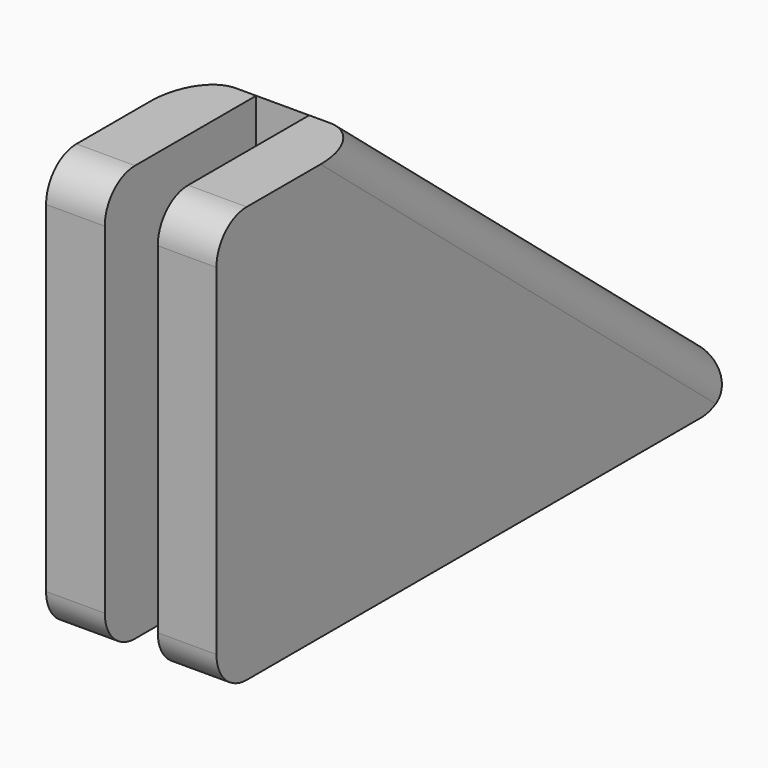
from build123d import *

# Parameters (mm, degrees)
F0_W     = 5
F0_H     = 10
F1_DEPTH = 4.5
F2_W     = 1.4
F2_H     = 5
F3_DEPTH = 25
F4_W     = 1.4
F4_H     = 1
F5_DEPTH = 25
F6_R     = 0.99999
F6_R_2   = 1
F7_R     = 5


# Not quite as in the source:
# - a fillet or chamfer is up to 0.001 mm smaller than in the source, because OpenCascade refuses the exact size


with BuildPart() as f1:
    # F0 (on Right) → F1 (new body)
    with BuildSketch(Plane.YZ):
        with Locations((-2.5, 5)):
            Rectangle(F0_W, F0_H)
        Polygon((0, 10), (0, 0), (12, 0), align=None)
        Polygon((12, 0), (0, 0), (-5, 0), (-5, -1), (12, -1), align=None)
    extrude(amount=F1_DEPTH)

    # F2 (on face) → F3 (cut)
    with BuildSketch(Plane.XY.offset(10)):
        with Locations((2.25, -2.5)):
            Rectangle(F2_W, F2_H)
    extrude(amount=-F3_DEPTH, mode=Mode.SUBTRACT)

    # F4 (on face) → F5 (cut)
    with BuildSketch(Plane(origin=(0, 12, 0), x_dir=(-1, 0, 0), z_dir=(0, 1, 0))):
        with Locations((-2.25, -0.5)):
            Rectangle(F4_W, F4_H)
    extrude(amount=-F5_DEPTH, mode=Mode.SUBTRACT)

    # F6 (call 1 of 8: OpenCascade refuses the feature's edges together) (radius 1 in the source; OpenCascade refuses exactly that, so slightly less here)
    f6_edges = [f1.edges().sort_by_distance(p)[0] for p in [
        (3.725, 12, -1),
    ]]
    fillet(f6_edges, radius=F6_R)

    # F6#2 (call 2 of 8) (radius 1 in the source; OpenCascade refuses exactly that, so slightly less here)
    f6_2_edges = [f1.edges().sort_by_distance(p)[0] for p in [
        (0.775, 12, -1),
    ]]
    fillet(f6_2_edges, radius=F6_R)

    # F6#3 (call 3 of 8)
    f6_3_edges = [f1.edges().sort_by_distance(p)[0] for p in [
        (3.725, -5, -1),
    ]]
    fillet(f6_3_edges, radius=F6_R_2)

    # F6#4 (call 4 of 8)
    f6_4_edges = [f1.edges().sort_by_distance(p)[0] for p in [
        (0.775, -5, -1),
    ]]
    fillet(f6_4_edges, radius=F6_R_2)

    # F6#5 (call 5 of 8)
    f6_5_edges = [f1.edges().sort_by_distance(p)[0] for p in [
        (0.775, -5, 10),
    ]]
    fillet(f6_5_edges, radius=F6_R_2)

    # F6#6 (call 6 of 8)
    f6_6_edges = [f1.edges().sort_by_distance(p)[0] for p in [
        (3.725, -5, 10),
    ]]
    fillet(f6_6_edges, radius=F6_R_2)

    # F6#7 (call 7 of 8)
    f6_7_edges = [f1.edges().sort_by_distance(p)[0] for p in [
        (0, 6, 5),
    ]]
    fillet(f6_7_edges, radius=F6_R_2)

    # F6#8 (call 8 of 8)
    f6_8_edges = [f1.edges().sort_by_distance(p)[0] for p in [
        (4.5, 6, 5),
    ]]
    fillet(f6_8_edges, radius=F6_R_2)

    # F7
    f7_edges = [f1.edges().sort_by_distance(p)[0] for p in [
        (2.25, 0, 0),
    ]]
    fillet(f7_edges, radius=F7_R)


solid = f1.part
